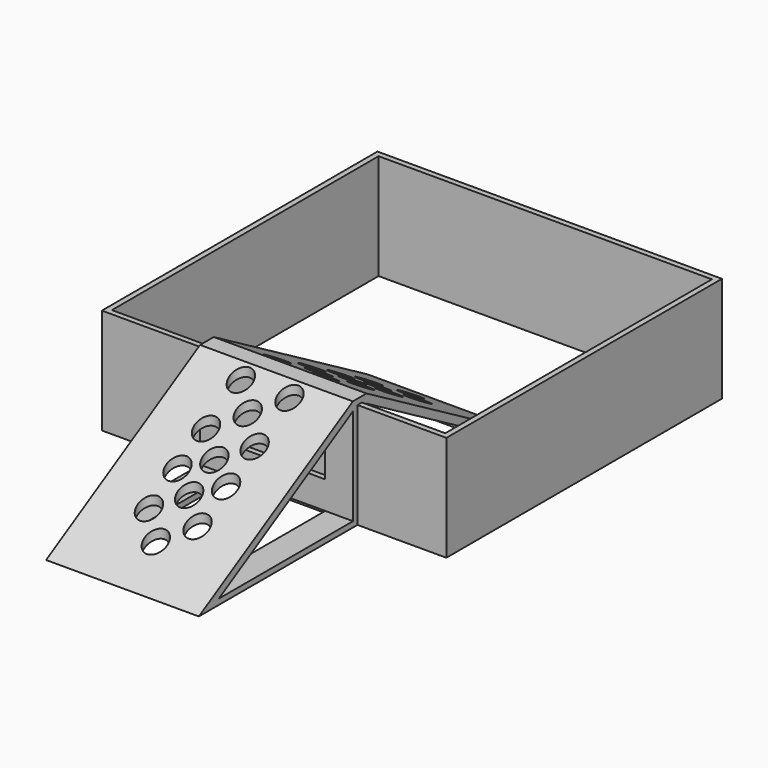
from build123d import *

# Parameters (mm, degrees)
F0_W          = 124
F0_H          = 124
F0_W_2        = 120
F0_H_2        = 120
F1_DEPTH      = 38
F2_W          = 2
F2_H          = 2
F3_DEPTH      = 30
F3_DEPTH_BACK = 25
F5_DEPTH      = 2
F6_R          = 4
F7_DEPTH      = 70
F8_W          = 35
F8_H          = 14.8452994616
F9_DEPTH      = 10


with BuildPart() as f1:
    # F0 (on Top) → F1 (new body)
    with BuildSketch(Plane.XY):
        Rectangle(F0_W, F0_H)
        Rectangle(F0_W_2, F0_H_2, mode=Mode.SUBTRACT)
    extrude(amount=F1_DEPTH)


with BuildPart() as f3:
    # F2 (on Right) → F3 (new body, two sides)
    with BuildSketch(Plane.YZ) as f3_sk:
        Polygon((-127.8179306876, 0), (-62, 0), (-62, 38), (-64, 36.8452994616), (-64, 38), (-64.0788376331, 38), (-64.0788376331, 40), (-133.3608699359, 0), align=None)
        Polygon((-124.3538290725, 2), (-64, 36.8452994616), (-64, 2), (-120.3538290725, 2), align=None, mode=Mode.SUBTRACT)
        Polygon((-64, 36.8452994616), (-62, 38), (-64, 38), align=None)
        Polygon((-64, 38), (-62, 38), (-62, 40), (-64.0788376331, 40), (-64.0788376331, 38), align=None)
        with Locations((-61, 39)):
            Rectangle(F2_W, F2_H)
        Polygon((-60, 40), (-60, 38), (-58, 36.8452994616), (-58, 38), (-57.9211623669, 40), align=None)
        Polygon((-58, 36.8452994616), (-60, 38), (-60, 0), (5.8179306876, 0), (11.3608699359, 0), (-57.9211623669, 40), (-58, 38), align=None)
        Polygon((-58, 2), (-58, 36.8452994616), (2.3538290725, 2), (-1.6461709275, 2), align=None, mode=Mode.SUBTRACT)
    extrude(amount=F3_DEPTH)
    extrude(f3_sk.sketch, amount=-F3_DEPTH_BACK)

    # F4 (on face) → F5 (cut)
    with BuildSketch(Plane(origin=(0, 0, 0), x_dir=(1, 0, 0), z_dir=(0, 0, -1))):
        Polygon((20, 123.3608699359), (-15, 123.3608699359), (-15, 72), (-15, 50), (-15, -1.3608699359), (-10.7783097774, -1.3608699359), (15.7783097774, -1.3608699359), (20, -1.3608699359), (20, 50), (20, 72), align=None)
    extrude(amount=-F5_DEPTH, mode=Mode.SUBTRACT)

    # F6 (on face) → F7 (cut)
    with BuildSketch(Plane(origin=(0, 0, 0), x_dir=(1, 0, 0), z_dir=(0, 0, -1))):
        with Locations((2.5, 118.3608699359)):
            Circle(F6_R)
        with Locations((2.5, 103.3608699359)):
            Circle(F6_R)
        with Locations((-6.25, 110.5206524519)):
            Circle(F6_R)
        with Locations((11.25, 110.5206524519)):
            Circle(F6_R)
        with Locations((2.5, 92)):
            Circle(F6_R)
        with Locations((11.25, 84.840217484)):
            Circle(F6_R)
        with Locations((2.5, 77)):
            Circle(F6_R)
        with Locations((-6.25, 84.840217484)):
            Circle(F6_R)
        with Locations((11.25, 69.159782516)):
            Circle(F6_R)
        with Locations((-6.25, 69.159782516)):
            Circle(F6_R)
        with Locations((11.25, 52.840217484)):
            Circle(F6_R)
        with Locations((2.5, 45)):
            Circle(F6_R)
        with Locations((-6.25, 52.840217484)):
            Circle(F6_R)
        with Locations((11.25, 37.159782516)):
            Circle(F6_R)
        with Locations((-6.25, 37.159782516)):
            Circle(F6_R)
        with Locations((2.5, 30)):
            Circle(F6_R)
        with Locations((2.5, 18.6391300641)):
            Circle(F6_R)
        with Locations((11.25, 11.4793475481)):
            Circle(F6_R)
        with Locations((2.5, 3.6391300641)):
            Circle(F6_R)
        with Locations((-6.25, 11.4793475481)):
            Circle(F6_R)
        with Locations((-6.25, 97.6804349679)):
            Circle(F6_R)
        with Locations((11.25, 97.6804349679)):
            Circle(F6_R)
        with Locations((-6.25, 24.3195650321)):
            Circle(F6_R)
        with Locations((11.25, 24.3195650321)):
            Circle(F6_R)
    extrude(amount=-F7_DEPTH, mode=Mode.SUBTRACT)

    # F8 (on face) → F9 (cut)
    with BuildSketch(Plane.XZ.offset(64)):
        with Locations((2.5, 19.4226497308)):
            Rectangle(F8_W, F8_H)
    extrude(amount=-F9_DEPTH, mode=Mode.SUBTRACT)


solid = Compound([f1.part, f3.part])
